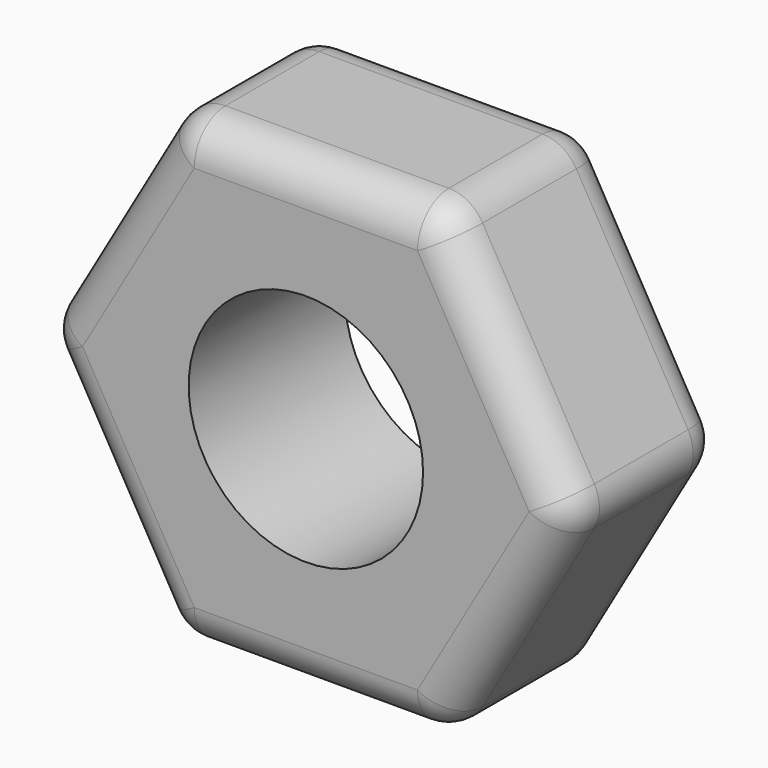
from build123d import *

# Parameters (mm, degrees)
F0_R     = 3
F1_DEPTH = 5
F2_R     = 1


# Not quite as in the source:
# - a feature names something its author has since deleted; it is built from what else it names


with BuildPart() as f1:
    # F0 (on Front) → F1 (new body)
    with BuildSketch(Plane.XZ):
        Polygon((-3.4352341017, 5.95), (-6.8704682034, 0), (-3.4352341017, -5.95), (3.4352341017, -5.95), (6.8704682034, 0), (3.4352341017, 5.95), align=None)
        Circle(F0_R, mode=Mode.SUBTRACT)
    extrude(amount=F1_DEPTH)

    # F2
    f2_edges = [f1.edges().sort_by_distance(p)[0] for p in [
        (-3.435234, -2.5, 5.95),
        (-6.870468, -2.5, 0),
        (-3.435234, -2.5, -5.95),
        (3.435234, -2.5, 5.95),
        (6.870468, -2.5, 0),
        (3.435234, -2.5, -5.95),
        (5.152851, -5, -2.975),
        (5.152851, 0, -2.975),
        (5.152851, 0, 2.975),
        (5.152851, -5, 2.975),
        (0, -5, -5.95),
        (0, 0, -5.95),
        (-5.152851, 0, -2.975),
        (-5.152851, -5, -2.975),
        (-5.152851, -5, 2.975),
        (0, -5, 5.95),
        (0, 0, 5.95),
        (-5.152851, 0, 2.975),
    ]]
    fillet(f2_edges, radius=F2_R)


solid = f1.part
